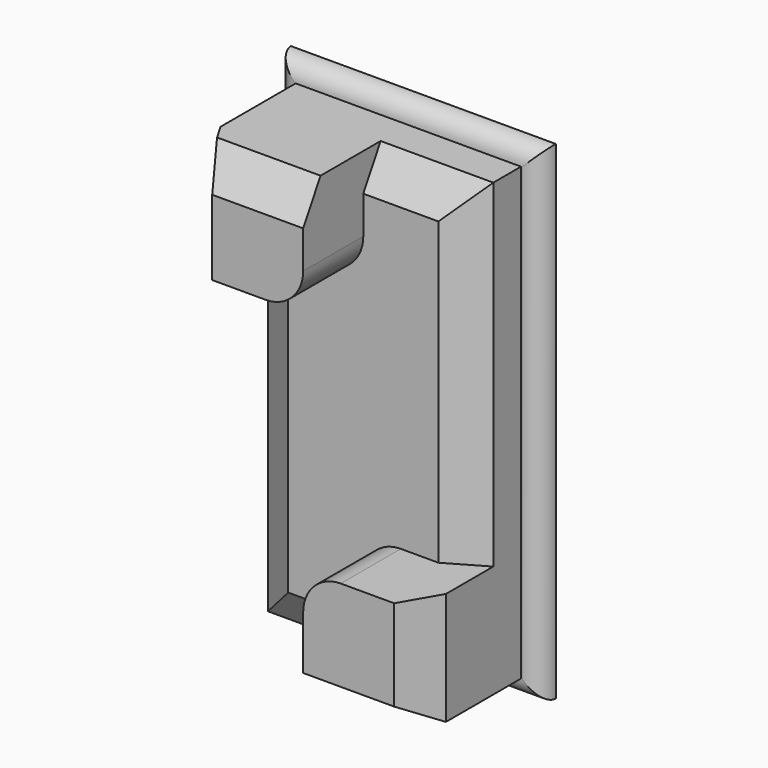
from build123d import *

# Parameters (mm, degrees)
F0_W        = 89.5588581535
F0_H        = 165.1
F1_DEPTH    = 6.35
F2_DEPTH    = 25.4
F3_DEPTH    = 50.8
F4_R        = 6.34999
F5_SIZE2    = 7.3323484187
F5_SIZE     = 12.7
F6_C1_SIZE2 = 7.3323484187
F6_C1_SIZE  = 12.7
F6_C2_SIZE2 = 7.3323484187
F6_C2_SIZE  = 12.7
F6_C3_SIZE2 = 12.7
F6_C3_SIZE  = 7.3323484187
F6_C4_SIZE2 = 7.3323484187
F6_C4_SIZE  = 12.7


# Not quite as in the source:
# - a fillet or chamfer is up to 0.001 mm smaller than in the source, because OpenCascade refuses the exact size


with BuildPart() as f1:
    # F0 (on Front) → F1 (new body)
    with BuildSketch(Plane.XZ):
        Rectangle(F0_W, F0_H)
        Polygon((-38.1, 38.1), (-38.1, 76.2), (0, 76.2), (38.1, 76.2), (38.1, -38.1), (38.1, -76.2), (0, -76.2), (-38.1, -76.2), align=None, mode=Mode.SUBTRACT)
    extrude(amount=F1_DEPTH)

    # F0 (on Front) → F2 (join)
    with BuildSketch(Plane.XZ):
        with BuildLine():
            Line((38.1, 76.2), (0, 76.2))
            Line((0, 76.2), (0, 50.8))
            ThreePointArc((0, 50.8), (-3.7197438789, 41.8197438789), (-12.7, 38.1))
            Line((-12.7, 38.1), (-38.1, 38.1))
            Line((-38.1, 38.1), (-38.1, -76.2))
            Line((-38.1, -76.2), (0, -76.2))
            Line((0, -76.2), (0, -50.8))
            ThreePointArc((0, -50.8), (3.7197438789, -41.8197438789), (12.7, -38.1))
            Line((12.7, -38.1), (38.1, -38.1))
            Line((38.1, -38.1), (38.1, 76.2))
        make_face()
    extrude(amount=F2_DEPTH)

    # F0 (on Front) → F3 (join)
    with BuildSketch(Plane.XZ):
        with BuildLine():
            Line((0, 76.2), (-38.1, 76.2))
            Line((-38.1, 76.2), (-38.1, 38.1))
            Line((-38.1, 38.1), (-12.7, 38.1))
            ThreePointArc((-12.7, 38.1), (-3.7197438789, 41.8197438789), (0, 50.8))
            Line((0, 50.8), (0, 76.2))
        make_face()
        with BuildLine():
            Line((38.1, -76.2), (38.1, -38.1))
            Line((38.1, -38.1), (12.7, -38.1))
            ThreePointArc((12.7, -38.1), (3.7197438789, -41.8197438789), (0, -50.8))
            Line((0, -50.8), (0, -76.2))
            Line((0, -76.2), (38.1, -76.2))
        make_face()
    extrude(amount=F3_DEPTH)

    # F4 (radius 6.35 in the source; OpenCascade refuses exactly that, so slightly less here)
    f4_edges = [f1.edges().sort_by_distance(p)[0] for p in [
        (-44.779429, -6.35, 0),
        (0, -6.35, 82.55),
        (0, -6.35, -82.55),
        (44.779429, -6.35, 0),
    ]]
    fillet(f4_edges, radius=F4_R)

    # F5
    f5_edges = [f1.edges().sort_by_distance(p)[0] for p in [
        (-19.05, -25.4, -76.2),
        (38.1, -25.4, 19.05),
        (-38.1, -25.4, -19.05),
        (19.05, -25.4, 76.2),
    ]]
    f5_side = f1.faces().sort_by_distance((0, -25.4, 0))[0]
    chamfer(f5_edges, length=F5_SIZE, length2=F5_SIZE2, reference=f5_side)

    # F6: chamfer of 12.7 x 7.3323484187 on 4 edges, made by hand

    # F6_c1
    f6_c1_edges = [f1.edges().sort_by_distance(p)[0] for p in [
        (-38.1, -50.8, 57.15),
    ]]
    f6_c1_side = f1.faces().sort_by_distance((-38.1, -50.6533530316, 57.15))[0]
    chamfer(f6_c1_edges, length=F6_C1_SIZE, length2=F6_C1_SIZE2, reference=f6_c1_side)

    # F6_c2
    f6_c2_edges = [f1.edges().sort_by_distance(p)[0] for p in [
        (19.05, -50.8, -76.2),
    ]]
    f6_c2_side = f1.faces().sort_by_distance((19.05, -50.6533530316, -76.2))[0]
    chamfer(f6_c2_edges, length=F6_C2_SIZE, length2=F6_C2_SIZE2, reference=f6_c2_side)

    # F6_c3
    f6_c3_edges = [f1.edges().sort_by_distance(p)[0] for p in [
        (-15.3838257906, -50.8, 76.2),
    ]]
    f6_c3_side = f1.faces().sort_by_distance((-15.3838257906, -50.6533530316, 76.2))[0]
    chamfer(f6_c3_edges, length=F6_C3_SIZE, length2=F6_C3_SIZE2, reference=f6_c3_side)

    # F6_c4
    f6_c4_edges = [f1.edges().sort_by_distance(p)[0] for p in [
        (38.1, -50.8, -53.4838257906),
    ]]
    f6_c4_side = f1.faces().sort_by_distance((38.1, -50.6533530316, -53.4838257906))[0]
    chamfer(f6_c4_edges, length=F6_C4_SIZE, length2=F6_C4_SIZE2, reference=f6_c4_side)


solid = f1.part
